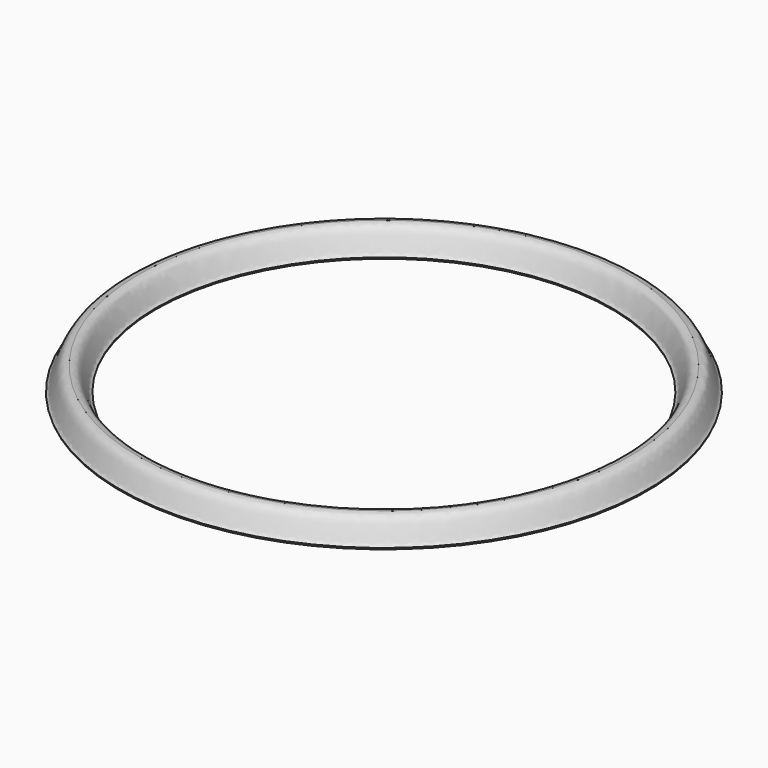
from build123d import *


# Not quite as in the source:
# - ends of sketch curves that miss each other by under 0.0002 mm in the source are joined
# - the dataset's text gives a spline's control points without its knots; the knots are read off the source's solid


with BuildPart() as f1:
    # F0 (on Front) → F1 (revolve)
    with BuildSketch(Plane.XZ):
        with BuildLine():
            add(Edge.make_bspline(
                [(-33.673491329, -10.746460408), (-30.2940776109, -9.5847869424), (-26.8487391771, -2.9517312884), (-16.1536775955, 30.6827537692), (-4.2565289879, 31.7319020918), (0, 32.1792960167)],
                knots=[0, 0, 0, 0, 0.253055809, 0.7058037164, 1, 1, 1, 1], degree=3))
            Line((-33.673491329, -10.746460408), (-32.6413630639, -13.7490153608))
            add(Edge.make_bspline(
                [(-32.6413630639, -13.7490153608), (-32.0962425463, -13.5616301828), (-31.046450311, -13.1228279851), (-29.6120656568, -12.2426857461), (-28.3639173439, -11.153963509), (-27.3246414028, -9.9131187607), (-26.4652990678, -8.5709945435), (-25.7289394786, -7.1428705696), (-25.0575509723, -5.6150665902), (-24.4034878727, -3.966461818), (-23.7200129331, -2.1586784961), (-22.7524429263, 0.4619432555), (-21.4390332444, 4.0527980839), (-19.6943876882, 8.6336541973), (-17.7893309715, 13.2331450383), (-15.7395466608, 17.5892727892), (-13.9354351571, 20.7874488056), (-12.4701363906, 22.9403819955), (-11.5589800124, 24.0859591421), (-10.8471405797, 24.8633535739), (-10.1479317433, 25.5477836542), (-8.9169623811, 26.5589629411), (-7.1366978466, 27.5610865699), (-4.8488431037, 28.3085620887), (-2.4596388179, 28.7268083984), (-0.7964342694, 28.9033245775), (2.8901e-06, 28.9868706605)],
                knots=[0, 0, 0, 0, 0.03125, 0.0625, 0.09375, 0.125, 0.15625, 0.1875, 0.21875, 0.25, 0.28125, 0.3125, 0.375, 0.4375, 0.5, 0.5625, 0.625, 0.65625, 0.6875, 0.703125, 0.71875, 0.75, 0.8125, 0.875, 0.9375, 0.9923987583, 0.9923987583, 0.9923987583, 0.9923987583], degree=3))
            add(Edge.make_bspline(
                [(32.6413630639, -13.7490153608), (32.0962425463, -13.5616301828), (31.046450311, -13.1228279851), (29.6120656568, -12.2426857461), (28.3639173439, -11.153963509), (27.3246414028, -9.9131187607), (26.4652990678, -8.5709945435), (25.7289394786, -7.1428705696), (25.0575509723, -5.6150665902), (24.4034878727, -3.966461818), (23.7200129331, -2.1586784961), (22.7524429263, 0.4619432555), (21.4390332444, 4.0527980839), (19.6943876882, 8.6336541973), (17.7893309715, 13.2331450383), (15.7395466608, 17.5892727892), (13.9354351571, 20.7874488056), (12.4701363906, 22.9403819955), (11.5589800124, 24.0859591421), (10.8471405797, 24.8633535739), (10.1479317433, 25.5477836542), (8.9169623811, 26.5589629411), (7.1366978466, 27.5610865699), (4.8488431037, 28.3085620887), (2.4596405625, 28.726808093), (0.7964379915, 28.9033241825), (2.8901e-06, 28.9868706605)],
                knots=[0, 0, 0, 0, 0.03125, 0.0625, 0.09375, 0.125, 0.15625, 0.1875, 0.21875, 0.25, 0.28125, 0.3125, 0.375, 0.4375, 0.5, 0.5625, 0.625, 0.65625, 0.6875, 0.703125, 0.71875, 0.75, 0.8125, 0.875, 0.9375, 0.9923986269, 0.9923986269, 0.9923986269, 0.9923986269], degree=3))
            Line((32.6413630639, -13.7490153608), (33.673491329, -10.746460408))
            add(Edge.make_bspline(
                [(33.673491329, -10.746460408), (30.2940776109, -9.5847869424), (26.8487391771, -2.9517312884), (16.1536775955, 30.6827537692), (4.2565289879, 31.7319020918), (0, 32.1792960167)],
                knots=[0, 0, 0, 0, 0.253055809, 0.7058037164, 1, 1, 1, 1], degree=3))
        make_face()
    revolve(axis=Axis((455.9867680073, 0, -19.4225162268), (0, 0, -1)))


solid = f1.part
